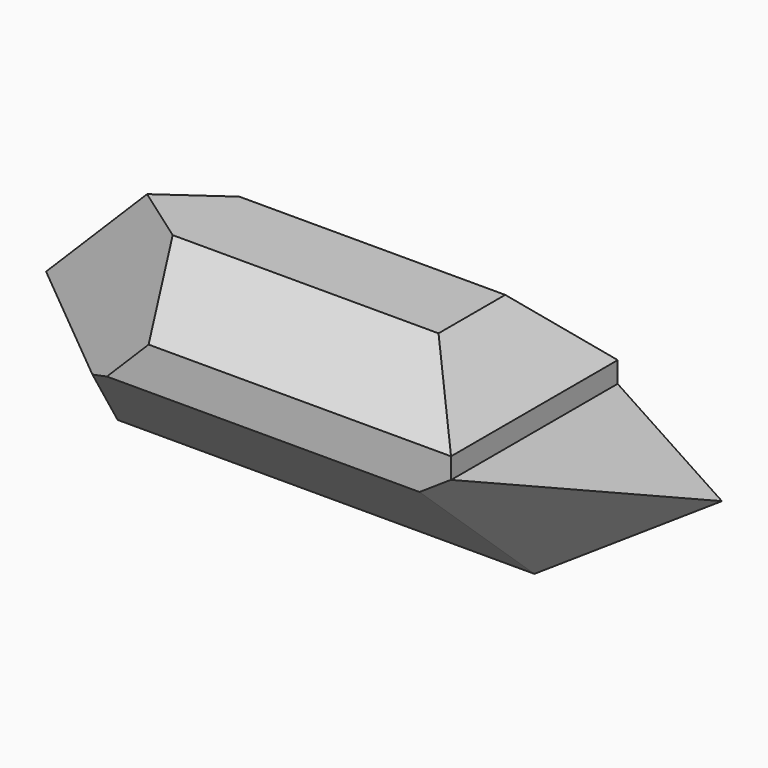
from build123d import *

# Parameters (mm, degrees)
F0_W         = 254
F0_H         = 76.2
F1_DEPTH     = 63.5
F2_SIZE      = 63.49999
F3_DEPTH     = 63.5
F4_T1_DEPTH  = 463.9752430668
F5_T1_DEPTH  = 463.9752430668
F6_DEPTH     = 63.5
F7_T1_DEPTH  = 418.1847418685
F0_H_2       = 50.8
F8_DEPTH     = 63.5
F9_SIZE      = 38.1
F10_DEPTH    = 63.5
F11_T1_DEPTH = 463.7665363346


# Not quite as in the source:
# - a fillet or chamfer that OpenCascade refuses, or shapes differently, is made with other operations: its cross-section is extruded or revolved along the edge and cut away or added
# - a fillet or chamfer is up to 0.001 mm smaller than in the source, because OpenCascade refuses the exact size


with BuildPart() as f1:
    # F0 (on Front) → F1 (new body, symmetric)
    with BuildSketch(Plane.XZ):
        with Locations((-33.6120952994, -22.0760072346)):
            Rectangle(F0_W, F0_H)
    extrude(amount=F1_DEPTH, both=True)

    # F2 (size 63.5 in the source; OpenCascade refuses exactly that, so slightly less here)
    f2_edges = [f1.edges().sort_by_distance(p)[0] for p in [
        (-33.612095, -63.5, -60.176007),
        (-33.612095, 63.5, -60.176007),
    ]]
    chamfer(f2_edges, length=F2_SIZE)

    # F0 (on Front) → F3 (join, symmetric)
    with BuildSketch(Plane.XZ):
        Polygon((207.6879047006, 16.0239927654), (93.3879047006, 16.0239927654), (93.3879047006, -60.1760072346), align=None)
    extrude(amount=F3_DEPTH, both=True)

    # F4: chamfer of 63.5 on 1 edges, made by hand

    # F4_s2 → F4_t1 (cut)
    with BuildSketch(Plane(origin=(-98.9957457875, 0, -65.9971638583), x_dir=(0, 1, 0), z_dir=(0.8320502943, 0, 0.5547001962))):
        Polygon((-63.5, -38.3717535941), (0, -101.8717535941), (-63.5, -101.8717535941), align=None)
    extrude(amount=F4_T1_DEPTH, mode=Mode.SUBTRACT)

    # F5: chamfer of 63.5 on 1 edges, made by hand

    # F5_s2 → F5_t1 (cut)
    with BuildSketch(Plane(origin=(-98.9957457875, 0, -65.9971638583), x_dir=(0, 1, 0), z_dir=(0.8320502943, 0, 0.5547001962))):
        Polygon((63.5, -38.3717535941), (0, -101.8717535941), (63.5, -101.8717535941), align=None)
    extrude(amount=F5_T1_DEPTH, mode=Mode.SUBTRACT)

    # F0 (on Front) → F6 (join, symmetric)
    with BuildSketch(Plane.XZ):
        Polygon((-160.6120952994, -60.1760072346), (-160.6120952994, 16.0239927654), (-211.4120952994, 16.0239927654), align=None)
    extrude(amount=F6_DEPTH, both=True)

    # F7: chamfer of 63.5 on 2 edges, made by hand

    # F7_s2 → F7_t1 (cut)
    with BuildSketch(Plane(origin=(-163.0291436318, 0, 244.5437154477), x_dir=(0, 1, 0), z_dir=(0.5547001962, 0, -0.8320502943))):
        Polygon((63.5, -103.5169841892), (0, -167.0169841892), (63.5, -167.0169841892), align=None)
        Polygon((-63.5, -103.5169841892), (0, -167.0169841892), (-63.5, -167.0169841892), align=None)
    extrude(amount=F7_T1_DEPTH, mode=Mode.SUBTRACT)

    # F0 (on Front) → F8 (join, symmetric)
    with BuildSketch(Plane.XZ):
        with Locations((-33.6120952994, 41.4239927654)):
            Rectangle(F0_W, F0_H_2)
    extrude(amount=F8_DEPTH, both=True)

    # F9
    f9_edges = [f1.edges().sort_by_distance(p)[0] for p in [
        (-33.612095, -63.5, 66.823993),
        (-33.612095, 63.5, 66.823993),
        (93.387905, 0, 66.823993),
    ]]
    chamfer(f9_edges, length=F9_SIZE)

    # F0 (on Front) → F10 (join, symmetric)
    with BuildSketch(Plane.XZ):
        Polygon((-211.4120952994, 16.0239927654), (-160.6120952994, 16.0239927654), (-160.6120952994, 66.8239927654), align=None)
    extrude(amount=F10_DEPTH, both=True)

    # F11: chamfer of 76.2 on 2 edges, made by hand

    # F11_s2 → F11_t1 (cut)
    with BuildSketch(Plane(origin=(91.6721800978, 0, 91.6721800978), x_dir=(0, 1, 0), z_dir=(-0.7071067812, 0, -0.7071067812))):
        Polygon((-63.5, -84.6216001572), (12.7, -160.8216001572), (-63.5, -160.8216001572), align=None)
        Polygon((63.5, -84.6216001572), (-12.7, -160.8216001572), (63.5, -160.8216001572), align=None)
    extrude(amount=F11_T1_DEPTH, mode=Mode.SUBTRACT)


solid = f1.part
